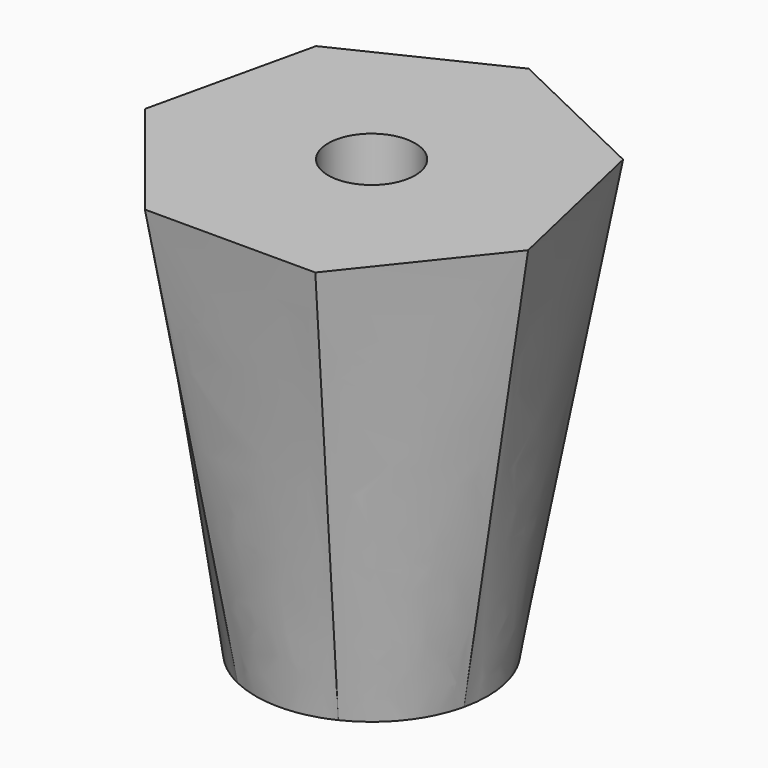
from build123d import *

# Parameters (mm, degrees)
F4_R     = 15
F5_DEPTH = 172


# Not quite as in the source:
# - the arcs of a loft's sections are written as splines that run evenly, so that the points pair up as in the source's solid


with BuildPart() as f3:
    # F1 (on Top) → F3 section 0
    with BuildSketch(Plane.XY):
        with BuildLine():
            add(Edge.make_bspline(
                [(31.2732592987, 24.9395920743), (28.7859564656, 28.0585711749), (25.8289364984, 30.8022847428), (19.2366681467, 35.2968172025), (15.6022965087, 37.0470383387), (7.9781174442, 39.3987861242), (3.9893240046, 40), (0, 40)],
                knots=[0, 0, 0, 0, 0.3333333333, 0.3333333333, 0.6666666667, 0.6666666667, 1, 1, 1, 1], degree=3))
            add(Edge.make_bspline(
                [(0, 40), (-3.9893240046, 40), (-7.9781174442, 39.3987861242), (-15.6022965087, 37.0470383387), (-19.2366681467, 35.2968172025), (-25.8289364984, 30.8022847428), (-28.7859564656, 28.0585711749), (-31.2732592987, 24.9395920743)],
                knots=[0, 0, 0, 0, 0.3333333333, 0.3333333333, 0.6666666667, 0.6666666667, 1, 1, 1, 1], degree=3))
            add(Edge.make_bspline(
                [(-31.2732592987, 24.9395920743), (-33.7605621319, 21.8206129738), (-35.7774862274, 18.3271979653), (-38.6924136641, 10.900083984), (-39.590029331, 6.967372789), (-40.1862744435, -0.9889653021), (-39.8848245906, -5.0115340355), (-38.9971164873, -8.9008373583)],
                knots=[0, 0, 0, 0, 0.3333333333, 0.3333333333, 0.6666666667, 0.6666666667, 1, 1, 1, 1], degree=3))
            add(Edge.make_bspline(
                [(-38.9971164873, -8.9008373583), (-38.1094083839, -12.790140681), (-36.6356781537, -16.5451440681), (-32.6463541491, -23.4548559319), (-30.1312909397, -26.6086454432), (-24.282528082, -32.0355043032), (-20.9496062968, -34.3078519004), (-17.3553495647, -36.0387547161)],
                knots=[0, 0, 0, 0, 0.3333333333, 0.3333333333, 0.6666666667, 0.6666666667, 1, 1, 1, 1], degree=3))
            add(Edge.make_bspline(
                [(-17.3553495647, -36.0387547161), (-13.7610928326, -37.7696575317), (-9.9064571986, -38.9586551589), (-2.0169240955, -40.1478109392), (2.0169240955, -40.1478109392), (9.9064571986, -38.9586551589), (13.7610928326, -37.7696575317), (17.3553495647, -36.0387547161)],
                knots=[0, 0, 0, 0, 0.3333333333, 0.3333333333, 0.6666666667, 0.6666666667, 1, 1, 1, 1], degree=3))
            add(Edge.make_bspline(
                [(17.3553495647, -36.0387547161), (20.9496062968, -34.3078519004), (24.282528082, -32.0355043032), (30.1312909397, -26.6086454432), (32.6463541491, -23.4548559319), (36.6356781537, -16.5451440681), (38.1094083839, -12.790140681), (38.9971164873, -8.9008373583)],
                knots=[0, 0, 0, 0, 0.3333333333, 0.3333333333, 0.6666666667, 0.6666666667, 1, 1, 1, 1], degree=3))
            add(Edge.make_bspline(
                [(38.9971164873, -8.9008373583), (39.8848245906, -5.0115340355), (40.1862744435, -0.9889653021), (39.590029331, 6.967372789), (38.6924136641, 10.900083984), (35.7774862274, 18.3271979653), (33.7605621319, 21.8206129738), (31.2732592987, 24.9395920743)],
                knots=[0, 0, 0, 0, 0.3333333333, 0.3333333333, 0.6666666667, 0.6666666667, 1, 1, 1, 1], degree=3))
        make_face()
    # F2 (on offset) → F3 section 1
    with BuildSketch(Plane.XY.offset(150)):
        Polygon((52.9471102464, 42.2239114397), (0, 67.7218958735), (-52.9471102464, 42.2239114397), (-66.023966553, -15.0695395191), (-29.3834294017, -61.0153198574), (29.3834294017, -61.0153198574), (66.023966553, -15.0695395191), align=None)
    loft(ruled=True)

    # F4 (on face) → F5 (cut)
    with BuildSketch(Plane(origin=(0, 0, 0), x_dir=(1, 0, 0), z_dir=(0, 0, -1))):
        Circle(F4_R)
    extrude(amount=-F5_DEPTH, mode=Mode.SUBTRACT)


solid = f3.part
